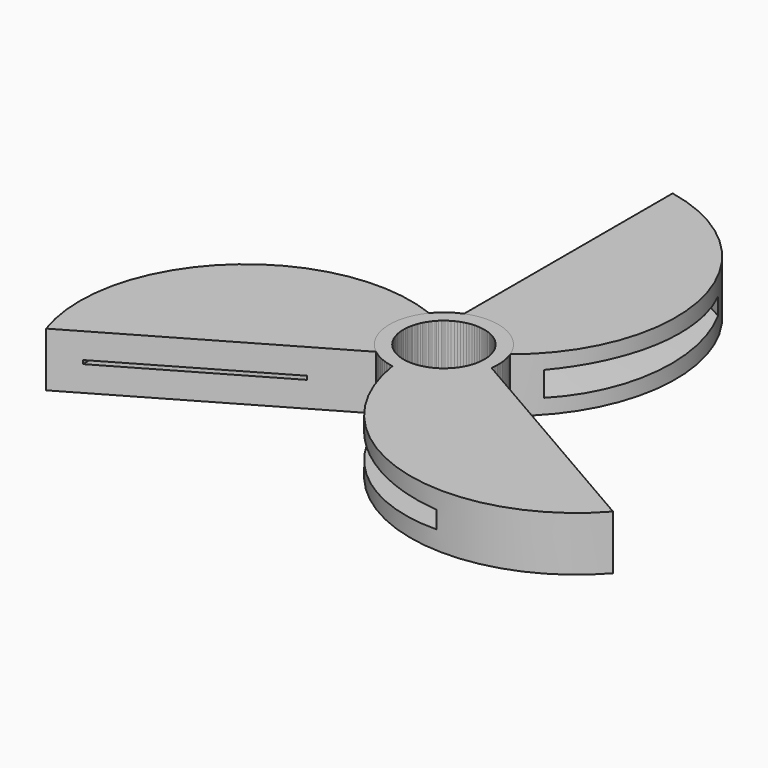
from build123d import *

# Parameters (mm, degrees)
F1_DEPTH = 15
F2_W     = 48.9160085236
F2_H     = 1
F5_W     = 49.5659764856
F5_H     = 7
F7_COUNT = 3


# Not quite as in the source:
# - a feature names something its author has since deleted; it is built from what else it names


with BuildPart() as f1:
    # F0 (on Top) → F1 (new body)
    with BuildSketch(Plane.XY):
        with BuildLine():
            Line((-9.272331311, -11.7908384799), (-5.575, -9.6561832522))
            ThreePointArc((-5.575, -9.6561832522), (-11.0484708107, -1.5012637164), (-7.9494537725, 7.8184835306))
            ThreePointArc((-7.9494537725, 7.8184835306), (-9.7808733397, 8.6754769013), (-11.6483927438, 9.4506585213))
            ThreePointArc((-11.6483927438, 9.4506585213), (-14.9070276198, -1.6674913921), (-9.272331311, -11.7908384799))
        make_face()
        with BuildLine():
            Line((-71.5661357684, -47.7561832522), (-9.272331311, -11.7908384799))
            ThreePointArc((-9.272331311, -11.7908384799), (-14.9070276198, -1.6674913921), (-11.6483927438, 9.4506585213))
            ThreePointArc((-11.6483927438, 9.4506585213), (-59.812015709, -0.0853294227), (-71.5661357684, -47.7561832522))
        make_face()
        with BuildLine():
            ThreePointArc((11.15, 0), (5.575, -9.6561832522), (-5.575, -9.6561832522))
            Line((-5.575, -9.6561832522), (-9.272331311, -11.7908384799))
            ThreePointArc((-9.272331311, -11.7908384799), (6.5541982856, -13.492312064), (15, 0))
            ThreePointArc((15, 0), (5.0136867095, 14.1372891878), (-11.6483927438, 9.4506585213))
            ThreePointArc((-11.6483927438, 9.4506585213), (-9.7808733397, 8.6754769013), (-7.9494537725, 7.8184835306))
            ThreePointArc((-7.9494537725, 7.8184835306), (4.2241028892, 10.3188882532), (11.15, 0))
        make_face()
    extrude(amount=F1_DEPTH)

    # F2 (on face) → F6 section 0
    with BuildSketch(Plane(origin=(2.7875, -4.8280916261, 0), x_dir=(0.8660254038, 0.5, 0), z_dir=(0.5, -0.8660254038, 0))):
        with Locations((-53.3981789904, 7.5)):
            Rectangle(F2_W, F2_H)
    # F5 (on offset) → F6 section 1
    with BuildSketch(Plane.XZ.offset(-12.7)):
        with Locations((-43.3189691976, 7.5000846907)):
            Rectangle(F5_W, F5_H)
    loft(mode=Mode.SUBTRACT)


with BuildPart() as f7_1:
    # F7: instance of F1
    add(f1.part.rotate(Axis((0, 0, 9.7341537476), (0, 0, -1)), 1 * 360 / F7_COUNT))


with BuildPart() as f7_2:
    # F7: instance of F1
    add(f1.part.rotate(Axis((0, 0, 9.7341537476), (0, 0, -1)), 2 * 360 / F7_COUNT))


solid = Compound([f1.part, f7_1.part, f7_2.part])
